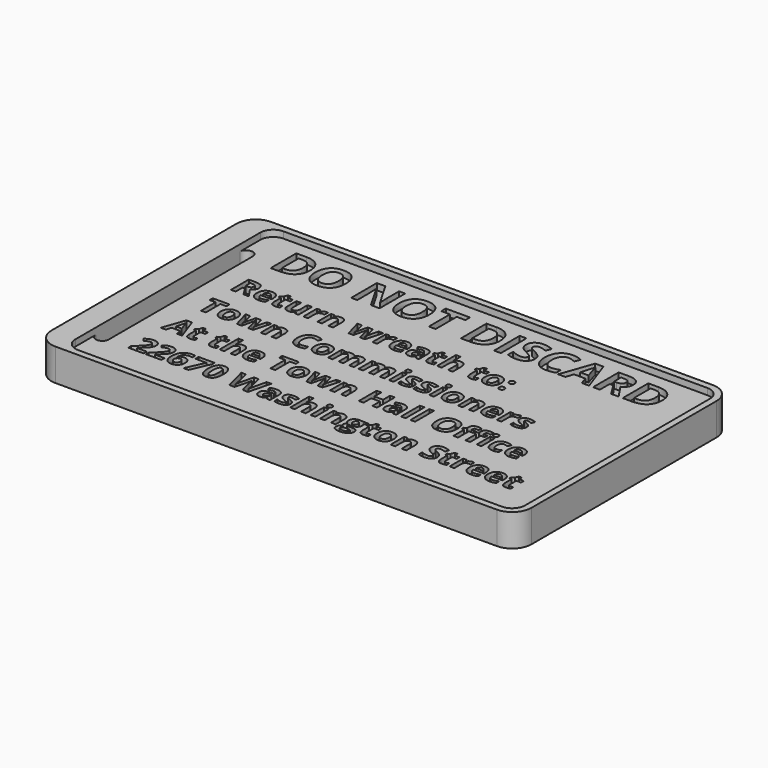
from build123d import *

# Parameters (mm, degrees)
F1_DEPTH       = 6.35
F2_DEPTH       = 5.08
F3_TEXT_SIZE   = 8.8599821957
F3_TEXT_SIZE_2 = 6.1334138243
F4_DEPTH       = 1.27


# Not quite as in the source:
# - Text() gives the source's letters only with a copy of the font that has no kerning and outlines rounded to 1/6400 em; it was checked with that copy


with BuildPart() as f1:
    # F0 (on Top) → F1 (new body)
    with BuildSketch(Plane.XY):
        with BuildLine():
            Line((-0.9129742631, -1.27), (2.8970257369, -1.27))
            Line((2.8970257369, -1.27), (86.36, -1.27))
            ThreePointArc((86.36, -1.27), (89.0540768363, -0.1540768363), (90.17, 2.54))
            Line((90.17, 2.54), (90.17, 48.26))
            ThreePointArc((90.17, 48.26), (89.1835421071, 50.8360700741), (86.7170257369, 52.0711948439))
            Line((86.7170257369, 52.0711948439), (2.8970257369, 52.0711948439))
            Line((2.8970257369, 52.0711948439), (-0.9129742631, 52.0711948439))
            ThreePointArc((-0.9129742631, 52.0711948439), (-3.6070510995, 50.9552716802), (-4.7229742631, 48.2611948439))
            Line((-4.7229742631, 48.2611948439), (-4.7229742631, 2.54))
            ThreePointArc((-4.7229742631, 2.54), (-3.6070510995, -0.1540768363), (-0.9129742631, -1.27))
        make_face()
        with BuildLine():
            Line((86.36, 0), (2.54, 0))
            ThreePointArc((2.54, 0), (0.7439487758, 0.7439487758), (0, 2.54))
            Line((0, 2.54), (0, 7.62))
            Line((0, 7.62), (0, 43.18))
            Line((0, 43.18), (0, 48.26))
            ThreePointArc((0, 48.26), (0.7439487758, 50.0560512242), (2.54, 50.8))
            Line((2.54, 50.8), (86.36, 50.8))
            ThreePointArc((86.36, 50.8), (88.1560512242, 50.0560512242), (88.9, 48.26))
            Line((88.9, 48.26), (88.9, 2.54))
            ThreePointArc((88.9, 2.54), (88.1560512242, 0.7439487758), (86.36, 0))
        make_face(mode=Mode.SUBTRACT)
    extrude(amount=F1_DEPTH)

    # F0 (on Top) → F2 (join)
    with BuildSketch(Plane.XY):
        with BuildLine():
            ThreePointArc((0, 2.54), (0.7439487758, 0.7439487758), (2.54, 0))
            Line((2.54, 0), (86.36, 0))
            ThreePointArc((86.36, 0), (88.1560512242, 0.7439487758), (88.9, 2.54))
            Line((88.9, 2.54), (88.9, 48.26))
            ThreePointArc((88.9, 48.26), (88.1560512242, 50.0560512242), (86.36, 50.8))
            Line((86.36, 50.8), (2.54, 50.8))
            ThreePointArc((2.54, 50.8), (0.7439487758, 50.0560512242), (0, 48.26))
            Line((0, 48.26), (0, 43.18))
            ThreePointArc((0, 43.18), (1.27, 44.45), (2.54, 43.18))
            Line((2.54, 43.18), (2.54, 25.4))
            Line((2.54, 25.4), (2.54, 7.62))
            ThreePointArc((2.54, 7.62), (1.27, 6.35), (0, 7.62))
            Line((0, 7.62), (0, 2.54))
        make_face()
    extrude(amount=F2_DEPTH)

    # F3 (on face) → F4 (cut)
    with BuildSketch(Plane.XY.offset(5.08)):
        with Locations((6.35, 41.8808128191)):
            Text('DO NOT DISCARD', F3_TEXT_SIZE, font='Open Sans', font_style=FontStyle.BOLD, text_align=(TextAlign.LEFT, TextAlign.BOTTOM))
        with Locations((6.35, 32.3847548656)):
            Text('Return wreath to:', F3_TEXT_SIZE_2, font='Open Sans', font_style=FontStyle.BOLD, text_align=(TextAlign.LEFT, TextAlign.BOTTOM))
        with Locations((6.35, 24.0433120645)):
            Text('Town Commissioners', F3_TEXT_SIZE_2, font='Open Sans', font_style=FontStyle.BOLD, text_align=(TextAlign.LEFT, TextAlign.BOTTOM))
        with Locations((6.35, 15.7018692634)):
            Text('At the Town Hall Office', F3_TEXT_SIZE_2, font='Open Sans', font_style=FontStyle.BOLD, text_align=(TextAlign.LEFT, TextAlign.BOTTOM))
        with Locations((6.35, 7.3604264623)):
            Text('22670 Washington Street', F3_TEXT_SIZE_2, font='Open Sans', font_style=FontStyle.BOLD, text_align=(TextAlign.LEFT, TextAlign.BOTTOM))
    extrude(amount=-F4_DEPTH, mode=Mode.SUBTRACT)


solid = f1.part
